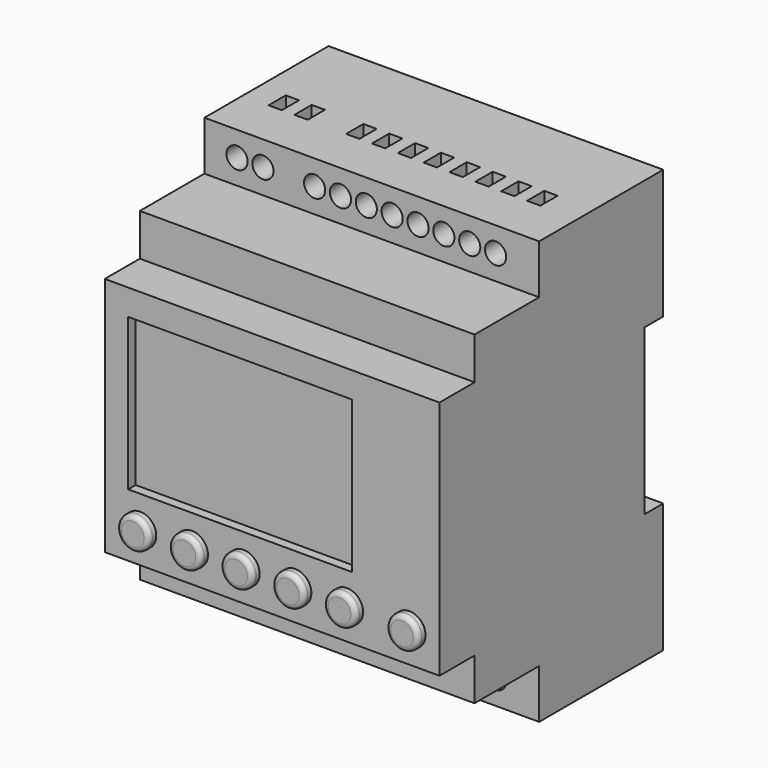
from build123d import *

# Parameters (mm, degrees)
F0_W      = 71.2
F0_H      = 90
F1_DEPTH  = 59.5
F2_W      = 5
F2_H      = 35
F3_DEPTH  = 71.2
F4_W      = 47.6332604885
F4_H      = 32.3030129075
F5_DEPTH  = 2
F4_R      = 3.4094371376
F4_R_2    = 3.409435
F6_DEPTH  = 2
F7_R      = 1
F8_R      = 2.25
F9_DEPTH  = 15
F10_W     = 2.8272345662
F10_H     = 4.5836474746
F11_DEPTH = 10
F12_W     = 2.8272345662
F12_H     = 4.5836474746
F13_DEPTH = 10


with BuildPart() as f1:
    # F0 (on Front) → F1 (new body)
    with BuildSketch(Plane.XZ):
        Rectangle(F0_W, F0_H)
    extrude(amount=F1_DEPTH)

    # F2 (on face) → F3 (cut, through all)
    with BuildSketch(Plane.YZ.offset(35.6)):
        Polygon((-33, 34.5271788538), (-33, 45), (-59.5, 45), (-59.5, 25.5845356733), (-50.1695893556, 25.5845356733), (-50.1695893556, 34.5271788538), align=None)
        Polygon((-50.1695893556, -25.5845356733), (-59.5, -25.5845356733), (-59.5, -45), (-33, -45), (-33, -34.5271788538), (-50.1695893556, -34.5271788538), align=None)
        with Locations((-2.5, 0)):
            Rectangle(F2_W, F2_H)
    extrude(amount=-F3_DEPTH, mode=Mode.SUBTRACT)

    # F4 (on face) → F5 (cut)
    with BuildSketch(Plane.XZ.offset(59.5)):
        with Locations((-6.800532341, 3.9449781179)):
            Rectangle(F4_W, F4_H)
    extrude(amount=-F5_DEPTH, mode=Mode.SUBTRACT)

    # F4 (on face) → F6 (join)
    with BuildSketch(Plane.XZ.offset(59.5)):
        with Locations((-28.0621219426, -18.9591366798)):
            Circle(F4_R)
        with Locations((-17.0621219426, -18.9591366798)):
            Circle(F4_R)
        with Locations((-6.0621219426, -18.9591366798)):
            Circle(F4_R)
        with Locations((4.9378780574, -18.9591366798)):
            Circle(F4_R)
        with Locations((15.9378780574, -18.9591366798)):
            Circle(F4_R)
        with Locations((29.2312186211, -18.9591366798)):
            Circle(F4_R_2)
    extrude(amount=F6_DEPTH)

    # F7
    f7_edges = [f1.edges().sort_by_distance(p)[0] for p in [
        (-31.471559, -61.5, -18.959137),
        (-20.471559, -61.5, -18.959137),
        (-9.471559, -61.5, -18.959137),
        (1.528441, -61.5, -18.959137),
        (12.528441, -61.5, -18.959137),
        (25.821784, -61.5, -18.959137),
    ]]
    fillet(f7_edges, radius=F7_R)

    # F8 (on face) → F9 (cut)
    with BuildSketch(Plane.XZ.offset(33)):
        with Locations((-28.6621302366, 39.7635894269)):
            Circle(F8_R)
        with Locations((-23.1621302366, 39.7635894269)):
            Circle(F8_R)
        with Locations((-12.1621302366, 39.7635894269)):
            Circle(F8_R)
        with Locations((-6.6621302366, 39.7635894269)):
            Circle(F8_R)
        with Locations((-1.1621302366, 39.7635894269)):
            Circle(F8_R)
        with Locations((4.3378697634, 39.7635894269)):
            Circle(F8_R)
        with Locations((9.8378697634, 39.7635894269)):
            Circle(F8_R)
        with Locations((15.3378697634, 39.7635894269)):
            Circle(F8_R)
        with Locations((20.8378697634, 39.7635894269)):
            Circle(F8_R)
        with Locations((26.3378697634, 39.7635894269)):
            Circle(F8_R)
        with Locations((-23.1621302366, -39.7635894269)):
            Circle(F8_R)
        with Locations((-28.6621302366, -39.7635894269)):
            Circle(F8_R)
        with Locations((-6.6621302366, -39.7635894269)):
            Circle(F8_R)
        with Locations((-12.1621302366, -39.7635894269)):
            Circle(F8_R)
        with Locations((26.3378697634, -39.7635894269)):
            Circle(F8_R)
        with Locations((20.8378697634, -39.7635894269)):
            Circle(F8_R)
        with Locations((9.8378697634, -39.7635894269)):
            Circle(F8_R)
        with Locations((4.3378697634, -39.7635894269)):
            Circle(F8_R)
    extrude(amount=-F9_DEPTH, mode=Mode.SUBTRACT)

    # F10 (on face) → F11 (cut)
    with BuildSketch(Plane.XY.offset(45)):
        with Locations((-28.6638047546, -20.5665649846)):
            Rectangle(F10_W, F10_H)
        with Locations((-23.1638047546, -20.5665649846)):
            Rectangle(F10_W, F10_H)
        with Locations((-12.1638047546, -20.5665649846)):
            Rectangle(F10_W, F10_H)
        with Locations((-6.6638047546, -20.5665649846)):
            Rectangle(F10_W, F10_H)
        with Locations((-1.1638047546, -20.5665649846)):
            Rectangle(F10_W, F10_H)
        with Locations((4.3361952454, -20.5665649846)):
            Rectangle(F10_W, F10_H)
        with Locations((9.8361952454, -20.5665649846)):
            Rectangle(F10_W, F10_H)
        with Locations((15.3361952454, -20.5665649846)):
            Rectangle(F10_W, F10_H)
        with Locations((20.8361952454, -20.5665649846)):
            Rectangle(F10_W, F10_H)
        with Locations((26.3361952454, -20.5665649846)):
            Rectangle(F10_W, F10_H)
    extrude(amount=-F11_DEPTH, mode=Mode.SUBTRACT)

    # F12 (on face) → F13 (cut)
    with BuildSketch(Plane(origin=(0, 0, -45), x_dir=(1, 0, 0), z_dir=(0, 0, -1))):
        with Locations((-28.6638047546, 20.5665649846)):
            Rectangle(F12_W, F12_H)
        with Locations((-23.1638047546, 20.5665649846)):
            Rectangle(F12_W, F12_H)
        with Locations((-12.1638047546, 20.5665649846)):
            Rectangle(F12_W, F12_H)
        with Locations((-6.6638047546, 20.5665649846)):
            Rectangle(F12_W, F12_H)
        with Locations((4.3361952454, 20.5665649846)):
            Rectangle(F12_W, F12_H)
        with Locations((9.8361952454, 20.5665649846)):
            Rectangle(F12_W, F12_H)
        with Locations((20.8361952454, 20.5665649846)):
            Rectangle(F12_W, F12_H)
        with Locations((26.3361952454, 20.5665649846)):
            Rectangle(F12_W, F12_H)
    extrude(amount=-F13_DEPTH, mode=Mode.SUBTRACT)


solid = f1.part
